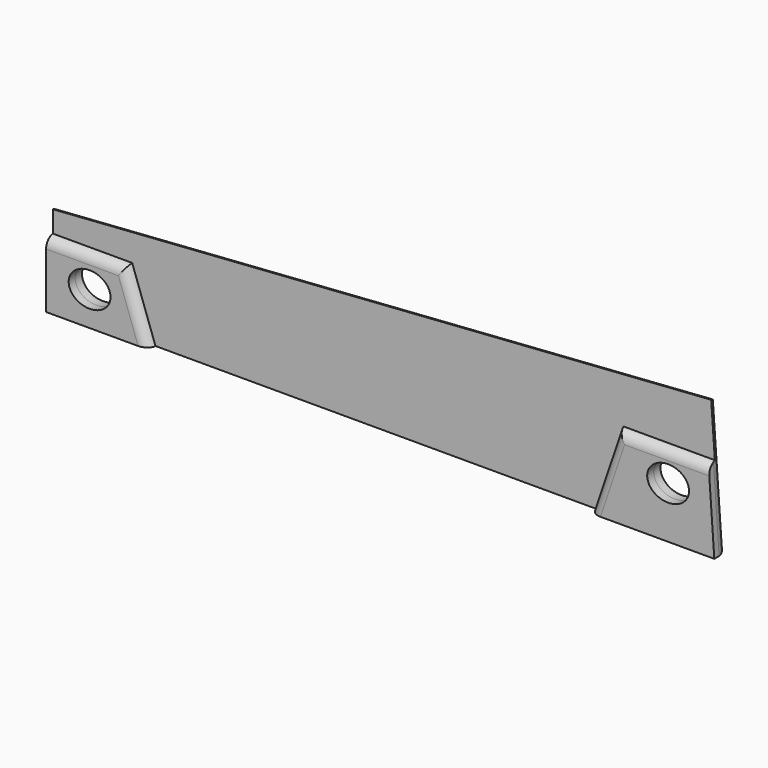
from build123d import *

# Parameters (mm, degrees)
F1_DEPTH    = 2.032
F3_DEPTH    = 1.9431
F4_T1_DEPTH = 34.2117387858
F4_T3_DEPTH = 32.9631500625
F4_T5_DEPTH = 31.3943412036
F4_T7_DEPTH = 29.0543755542
F5_T1_DEPTH = 170.4772089408
F5_T3_DEPTH = 44.7512757542
F5_T5_DEPTH = 172.5948607759
F5_T7_DEPTH = 33.5710337173


# Not quite as in the source:
# - a fillet or chamfer that OpenCascade refuses, or shapes differently, is made with other operations: its cross-section is extruded or revolved along the edge and cut away or added


with BuildPart() as f1:
    # F0 (on Front) → F1 (new body)
    with BuildSketch(Plane.XZ):
        Polygon((68.8549770113, 13.6631544467), (-88.7884451733, 2.5620862353), (-88.7884451733, -18.308947482), (71.1064156026, -18.308947482), align=None)
        with BuildLine():
            add(Edge.make_bspline(
                [(-73.3706451733, -10.180947482), (-73.3706451733, -3.141893), (-80.8763451733, -6.661420241), (-88.3820451733, -10.180947482), (-80.8763451733, -13.7004747229), (-73.3706451733, -17.2200019639), (-73.3706451733, -10.180947482)],
                knots=[0, 0, 0, 2.0943951024, 2.0943951024, 4.1887902048, 4.1887902048, 6.2831853072, 6.2831853072, 6.2831853072], degree=2, weights=[1, 0.5, 1, 0.5, 1, 0.5, 1]))
        make_face(mode=Mode.SUBTRACT)
        with BuildLine():
            add(Edge.make_bspline(
                [(65.0593548267, -6.015347482), (65.0593548267, 1.023707), (57.5536548267, -2.495820241), (50.0479548267, -6.015347482), (57.5536548267, -9.5348747229), (65.0593548267, -13.0544019639), (65.0593548267, -6.015347482)],
                knots=[0, 0, 0, 2.0943951024, 2.0943951024, 4.1887902048, 4.1887902048, 6.2831853072, 6.2831853072, 6.2831853072], degree=2, weights=[1, 0.5, 1, 0.5, 1, 0.5, 1]))
        make_face(mode=Mode.SUBTRACT)
    extrude(amount=F1_DEPTH)

    # F2 (on face) → F3 (join)
    with BuildSketch(Plane.XZ.offset(2.032)):
        Polygon((-88.7884451733, -18.308947482), (-64.1504451733, -18.308947482), (-69.7384451733, -2.560947482), (-88.7884451733, -2.560947482), align=None)
        with BuildLine():
            add(Edge.make_bspline(
                [(-73.3706451733, -10.180947482), (-73.3706451733, -3.141893), (-80.8763451733, -6.661420241), (-88.3820451733, -10.180947482), (-80.8763451733, -13.7004747229), (-73.3706451733, -17.2200019639), (-73.3706451733, -10.180947482)],
                knots=[0, 0, 0, 2.0943951024, 2.0943951024, 4.1887902048, 4.1887902048, 6.2831853072, 6.2831853072, 6.2831853072], degree=2, weights=[1, 0.5, 1, 0.5, 1, 0.5, 1]))
        make_face(mode=Mode.SUBTRACT)
        Polygon((47.8635548267, 1.223652518), (41.2595548267, -18.308947482), (71.1064156026, -18.308947482), (69.7309524089, 1.223652518), align=None)
        with BuildLine():
            add(Edge.make_bspline(
                [(65.0593548267, -6.015347482), (65.0593548267, 1.023707), (57.5536548267, -2.495820241), (50.0479548267, -6.015347482), (57.5536548267, -9.5348747229), (65.0593548267, -13.0544019639), (65.0593548267, -6.015347482)],
                knots=[0, 0, 0, 2.0943951024, 2.0943951024, 4.1887902048, 4.1887902048, 6.2831853072, 6.2831853072, 6.2831853072], degree=2, weights=[1, 0.5, 1, 0.5, 1, 0.5, 1]))
        make_face(mode=Mode.SUBTRACT)
    extrude(amount=F3_DEPTH)

    # F4: fillet of radius 2.54 on 4 edges, made by hand

    # F4_s2 → F4_t1 (cut)
    with BuildSketch(Plane.YZ.offset(41.6913842249)):
        with BuildLine():
            ThreePointArc((-2.032, 1.223652518), (-3.431061673, 0.3256875207), (-3.9751, -1.2452157227))
            Line((-3.9751, -1.2452157227), (-3.9751, 1.223652518))
            Line((-3.9751, 1.223652518), (-2.032, 1.223652518))
        make_face()
    extrude(amount=F4_T1_DEPTH, mode=Mode.SUBTRACT)

    # F4_s4 → F4_t3 (cut)
    with BuildSketch(Plane(origin=(7.2582801254, 0, 21.4677592939), x_dir=(0, 1, 0), z_dir=(-0.320290083, 0, -0.9473195146))):
        with BuildLine():
            ThreePointArc((-2.032, 44.9501557593), (-3.431061673, 45.8481207566), (-3.9751, 47.419024))
            Line((-3.9751, 47.419024), (-3.9751, 44.9501557593))
            Line((-3.9751, 44.9501557593), (-2.032, 44.9501557593))
        make_face()
    extrude(amount=F4_T3_DEPTH, mode=Mode.SUBTRACT)

    # F4_s6 → F4_t5 (cut)
    with BuildSketch(Plane.YZ.offset(-94.9606157751)):
        with BuildLine():
            ThreePointArc((-3.9751, -5.0298157227), (-3.431061673, -3.4589124793), (-2.032, -2.560947482))
            Line((-2.032, -2.560947482), (-3.9751, -2.560947482))
            Line((-3.9751, -2.560947482), (-3.9751, -5.0298157227))
        make_face()
    extrude(amount=F4_T5_DEPTH, mode=Mode.SUBTRACT)

    # F4_s8 → F4_t7 (cut)
    with BuildSketch(Plane(origin=(0.6602889826, 0, -1.8608144054), x_dir=(0, 1, 0), z_dir=(-0.3344098452, 0, 0.9424277455))):
        with BuildLine():
            ThreePointArc((-3.9751, 69.0487199497), (-3.431061673, 67.4778167063), (-2.032, 66.579851709))
            Line((-2.032, 66.579851709), (-3.9751, 66.579851709))
            Line((-3.9751, 66.579851709), (-3.9751, 69.0487199497))
        make_face()
    extrude(amount=F4_T7_DEPTH, mode=Mode.SUBTRACT)

    # F5: fillet of radius 2.54 on 4 edges, made by hand

    # F5_s2 → F5_t1 (cut)
    with BuildSketch(Plane(origin=(75.678953748, 0, 5.3292247535), x_dir=(0, 1, 0), z_dir=(-0.9975297762, 0, -0.0702448979))):
        with BuildLine():
            ThreePointArc((0, -6.3040109916), (-0.5725244601, -7.910448043), (-2.032, -8.7926925703))
            Line((-2.032, -8.7926925703), (0, -8.7926925703))
            Line((0, -8.7926925703), (0, -6.3040109916))
        make_face()
    extrude(amount=F5_T1_DEPTH, mode=Mode.SUBTRACT)

    # F5_s4 → F5_t3 (cut)
    with BuildSketch(Plane(origin=(2.0798519012, 0, -29.5354433558), x_dir=(0, 1, 0), z_dir=(-0.0702448979, 0, 0.9975297762))):
        with BuildLine():
            ThreePointArc((-2.54, -69.644656694), (-0.7439487758, -68.9007079182), (0, -67.104656694))
            Line((0, -67.104656694), (0, -69.644656694))
            Line((0, -69.644656694), (-2.54, -69.644656694))
        make_face()
    extrude(amount=F5_T3_DEPTH, mode=Mode.SUBTRACT)

    # F5_s6 → F5_t5 (cut)
    with BuildSketch(Plane.YZ.offset(-95.1384451733)):
        with BuildLine():
            ThreePointArc((-2.54, -18.308947482), (-0.7439487758, -17.5649987062), (0, -15.768947482))
            Line((0, -15.768947482), (0, -18.308947482))
            Line((0, -18.308947482), (-2.54, -18.308947482))
        make_face()
    extrude(amount=F5_T5_DEPTH, mode=Mode.SUBTRACT)

    # F5_s8 → F5_t7 (cut)
    with BuildSketch(Plane.XY.offset(-24.658947482)):
        with BuildLine():
            ThreePointArc((-86.2484451733, 0), (-88.0444963975, -0.7439487758), (-88.7884451733, -2.54))
            Line((-88.7884451733, -2.54), (-88.7884451733, 0))
            Line((-88.7884451733, 0), (-86.2484451733, 0))
        make_face()
    extrude(amount=F5_T7_DEPTH, mode=Mode.SUBTRACT)


solid = f1.part
